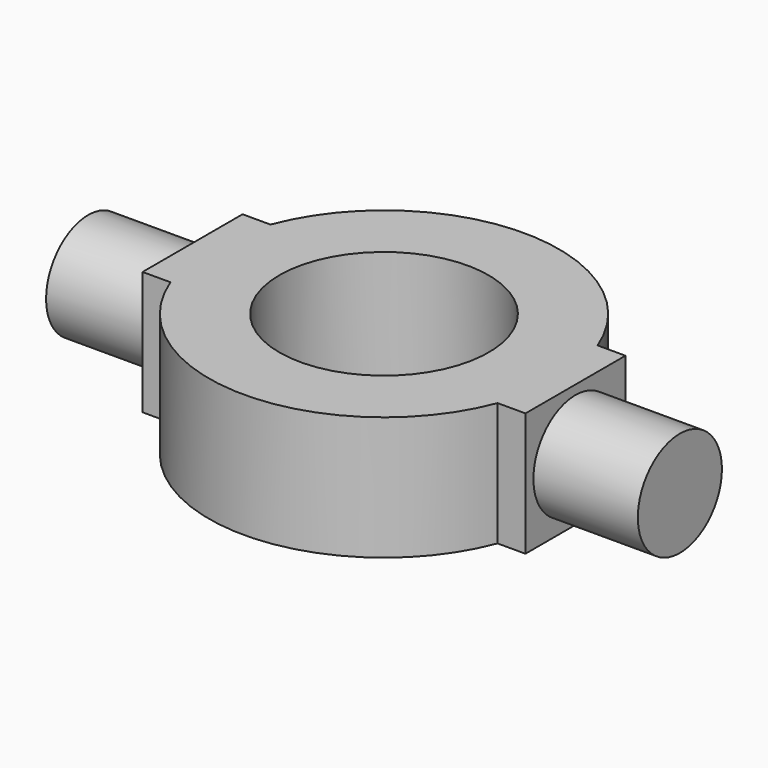
from build123d import *

# Parameters (mm, degrees)
F1_DEPTH = 17.75
F3_R     = 15.1
F4_DEPTH = 30
F6_R     = 15.1
F7_DEPTH = 30
F10_D    = 60.1


with BuildPart() as f1:
    # F0 (on Top) → F1 (new body, symmetric)
    with BuildSketch(Plane.XY):
        with BuildLine():
            ThreePointArc((46.9881634031, -17.95), (49.4651120446, -9.1264829157), (50.3, 0))
            ThreePointArc((50.3, 0), (49.4651120446, 9.1264829157), (46.9881634031, 17.95))
            Line((46.9881634031, 17.95), (-46.9881634031, 17.95))
            ThreePointArc((-46.9881634031, 17.95), (-50.3, 0), (-46.9881634031, -17.95))
            Line((-46.9881634031, -17.95), (46.9881634031, -17.95))
        make_face()
        with BuildLine():
            Line((-46.9881634031, 17.95), (46.9881634031, 17.95))
            ThreePointArc((46.9881634031, 17.95), (0, 50.3), (-46.9881634031, 17.95))
        make_face()
        with BuildLine():
            ThreePointArc((46.9881634031, 17.95), (49.4651120446, 9.1264829157), (50.3, 0))
            ThreePointArc((50.3, 0), (49.4651120446, -9.1264829157), (46.9881634031, -17.95))
            Line((46.9881634031, -17.95), (55, -17.95))
            Line((55, -17.95), (55, 17.95))
            Line((55, 17.95), (46.9881634031, 17.95))
        make_face()
        with BuildLine():
            ThreePointArc((-46.9881634031, -17.95), (0, -50.3), (46.9881634031, -17.95))
            Line((46.9881634031, -17.95), (-46.9881634031, -17.95))
        make_face()
        with BuildLine():
            ThreePointArc((-46.9881634031, -17.95), (-50.3, 0), (-46.9881634031, 17.95))
            Line((-46.9881634031, 17.95), (-55, 17.95))
            Line((-55, 17.95), (-55, -17.95))
            Line((-55, -17.95), (-46.9881634031, -17.95))
        make_face()
    extrude(amount=F1_DEPTH, both=True)

    # F3 (on offset) → F4 (join)
    with BuildSketch(Plane.YZ.offset(55)):
        Circle(F3_R)
    extrude(amount=F4_DEPTH)

    # F6 (on offset) → F7 (join)
    with BuildSketch(Plane(origin=(-55, 0, 0), x_dir=(0, -1, 0), z_dir=(-1, 0, 0))):
        Circle(F6_R)
    extrude(amount=F7_DEPTH)

    # F10 (through all)
    with Locations(Plane(origin=(0, 0, -17.75), x_dir=(1, 0, 0), z_dir=(0, 0, -1))):
        with Locations((0, 0)):
            Hole(F10_D / 2)


solid = f1.part
